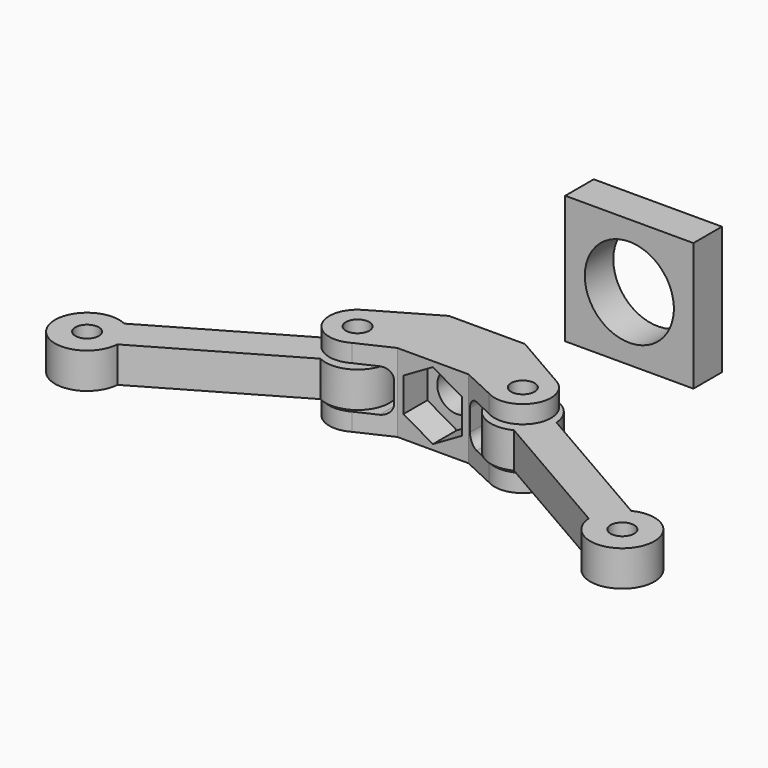
from build123d import *

# Parameters (mm, degrees)
F0_R      = 3.3
F1_DEPTH  = 22
F2_R      = 5.5
F3_DEPTH  = 18.9697660486
F4_R      = 5.5
F5_DEPTH  = 8.4
F6_W      = 29.9312670497
F6_H      = 12
F7_DEPTH  = 24.3375766425
F8_R      = 3
F10_R     = 3.3
F11_DEPTH = 10
F14_W     = 36
F14_H     = 36
F14_R     = 12.5
F15_DEPTH = 10


with BuildPart() as f1:
    # F0 (on Top) → F1 (new body)
    with BuildSketch(Plane.XY):
        with BuildLine():
            Line((10.6705042752, 0), (0, 0))
            Line((0, 0), (-10.6705042752, 0))
            Line((-10.6705042752, 0), (-27.1682882173, -9.525))
            ThreePointArc((-27.1682882173, -9.525), (-30.0736148598, -20.3678266425), (-19.2307882173, -23.2731532851))
            Line((-19.2307882173, -23.2731532851), (-10, -18.9687660486))
            Line((-10, -18.9687660486), (0, -18.9687660486))
            Line((0, -18.9687660486), (10, -18.9687660486))
            Line((10, -18.9687660486), (19.2307882173, -23.2731532851))
            ThreePointArc((19.2307882173, -23.2731532851), (30.0736148598, -20.3678266425), (27.1682882173, -9.525))
            Line((27.1682882173, -9.525), (10.6705042752, 0))
        make_face()
        with Locations((-23.1995382173, -16.3990766425)):
            Circle(F0_R, mode=Mode.SUBTRACT)
        with Locations((23.1995382173, -16.3990766425)):
            Circle(F0_R, mode=Mode.SUBTRACT)
    extrude(amount=F1_DEPTH)

    # F2 (on face) → F3 (cut, through all)
    with BuildSketch(Plane.XZ.offset(18.9687660486)):
        with Locations((0, 11)):
            Circle(F2_R)
    extrude(amount=-F3_DEPTH, mode=Mode.SUBTRACT)

    # F4 (on face) → F5 (cut)
    with BuildSketch(Plane.XZ.offset(18.9687660486)):
        Polygon((-8.25, 15.7631397208), (-8.25, 6.2368602792), (0, 1.4737205584), (8.25, 6.2368602792), (8.25, 15.7631397208), (0, 20.5262794416), align=None)
        with Locations((0, 11)):
            Circle(F4_R, mode=Mode.SUBTRACT)
    extrude(amount=-F5_DEPTH, mode=Mode.SUBTRACT)

    # F6 (on face) → F7 (cut, through all)
    with BuildSketch(Plane(origin=(0, 0, 0), x_dir=(-1, 0, 0), z_dir=(0, 1, 0))):
        with Locations((-25.6361378, 11)):
            Rectangle(F6_W, F6_H)
        with Locations((25.6361378, 11)):
            Rectangle(F6_W, F6_H)
    extrude(amount=-F7_DEPTH, mode=Mode.SUBTRACT)

    # F8
    f8_edges = [f1.edges().sort_by_distance(p)[0] for p in [
        (10.670504, -9.640714, 5),
        (10.670504, -9.640714, 17),
        (-10.670504, -9.640714, 17),
        (-10.670504, -9.640714, 5),
    ]]
    fillet(f8_edges, radius=F8_R)


with BuildPart() as f11:
    # F10 (on offset) → F11 (new body)
    with BuildSketch(Plane.XY.offset(6)):
        with BuildLine():
            Line((71.1803217459, -38.3272922368), (32.1802789157, -15.8106070104))
            ThreePointArc((32.1802789157, -15.8106070104), (15.4053095832, -11.8990766425), (27.1802789157, -24.4708610482))
            Line((27.1802789157, -24.4708610482), (66.1803217459, -46.9875462747))
            ThreePointArc((66.1803217459, -46.9875462747), (82.9552910784, -50.8990766425), (71.1803217459, -38.3272922368))
        make_face()
        with Locations((75.1610624444, -46.3990766425)):
            Circle(F10_R, mode=Mode.SUBTRACT)
        with Locations((23.1995382173, -16.3990766425)):
            Circle(F10_R, mode=Mode.SUBTRACT)
    extrude(amount=F11_DEPTH)


with BuildPart() as f12_1:
    # F12: instance of F11
    add(f11.part.mirror(Plane.YZ))


with BuildPart() as f15:
    # F14 (on offset) → F15 (new body)
    with BuildSketch(Plane(origin=(0, 50, 0), x_dir=(-1, 0, 0), z_dir=(0, 1, 0))):
        with Locations((0, 11)):
            Rectangle(F14_W, F14_H)
        with Locations((0, 11)):
            Circle(F14_R, mode=Mode.SUBTRACT)
    extrude(amount=F15_DEPTH)


solid = Compound([f1.part, f11.part, f12_1.part, f15.part])
